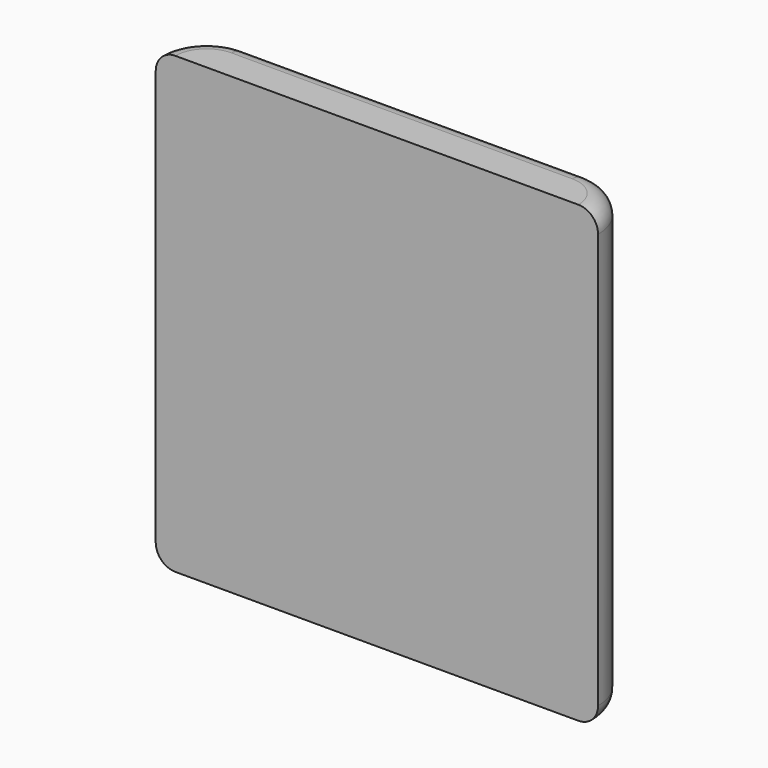
from build123d import *

# Parameters (mm, degrees)
F0_W         = 495.8
F0_H         = 57
F1_DEPTH     = 509.2
F2_R         = 56.99999
F3_T1_DEPTH  = 381.80002
F3_T3_DEPTH  = 55.00001
F3_T6_ANGLE  = 90
F3_T8_ANGLE  = 90
F3_T10_ANGLE = 90
F3_T12_ANGLE = 90


# Not quite as in the source:
# - a fillet or chamfer that OpenCascade refuses, or shapes differently, is made with other operations: its cross-section is extruded or revolved along the edge and cut away or added
# - a fillet or chamfer is up to 0.001 mm smaller than in the source, because OpenCascade refuses the exact size


with BuildPart() as f1:
    # F0 (on Top) → F1 (new body)
    with BuildSketch(Plane.XY):
        with Locations((247.9, 28.5)):
            Rectangle(F0_W, F0_H)
    extrude(amount=-F1_DEPTH)

    # F2 (radius 57 in the source; OpenCascade refuses exactly that, so slightly less here)
    f2_edges = [f1.edges().sort_by_distance(p)[0] for p in [
        (495.8, 57, -254.6),
        (0, 57, -254.6),
    ]]
    fillet(f2_edges, radius=F2_R)

    # F3: fillet of radius 22 on 6 edges, made by hand

    # F3_s2 → F3_t1 (cut)
    with BuildSketch(Plane.YZ.offset(56.99999)):
        with BuildLine():
            ThreePointArc((35, 0), (50.5563491861, -6.4436508139), (57, -22))
            Line((57, -22), (57, 0))
            Line((57, 0), (35, 0))
        make_face()
        with BuildLine():
            ThreePointArc((35, -509.2), (50.5563491861, -502.7563491861), (57, -487.2))
            Line((57, -487.2), (57, -509.2))
            Line((57, -509.2), (35, -509.2))
        make_face()
    extrude(amount=F3_T1_DEPTH, mode=Mode.SUBTRACT)

    # F3_s4 → F3_t3 (cut)
    with BuildSketch(Plane.XZ.offset(-1e-05)):
        with BuildLine():
            ThreePointArc((473.8, -509.2), (489.3563491861, -502.7563491861), (495.8, -487.2))
            Line((495.8, -487.2), (495.8, -509.2))
            Line((495.8, -509.2), (473.8, -509.2))
        make_face()
        with BuildLine():
            ThreePointArc((0, -487.2), (6.4436508139, -502.7563491861), (22, -509.2))
            Line((22, -509.2), (0, -509.2))
            Line((0, -509.2), (0, -487.2))
        make_face()
        with BuildLine():
            ThreePointArc((0, -22), (6.4436508139, -6.4436508139), (22, 0))
            Line((22, 0), (0, 0))
            Line((0, 0), (0, -22))
        make_face()
        with BuildLine():
            ThreePointArc((473.8, 0), (489.3563491861, -6.4436508139), (495.8, -22))
            Line((495.8, -22), (495.8, 0))
            Line((495.8, 0), (473.8, 0))
        make_face()
    extrude(amount=F3_T3_DEPTH, mode=Mode.SUBTRACT)

    # F3_s5 → F3_t6 (revolve, cut)
    with BuildSketch(Plane.XZ.offset(-1e-05)):
        with BuildLine():
            ThreePointArc((473.8, 0), (489.3563491861, -6.4436508139), (495.8, -22))
            Line((495.8, -22), (495.8, 0))
            Line((495.8, 0), (473.8, 0))
        make_face()
    revolve(axis=Axis((438.80001, 1e-05, 0), (0, 0, 1)), revolution_arc=F3_T6_ANGLE, mode=Mode.SUBTRACT)

    # F3_s7 → F3_t8 (revolve, cut)
    with BuildSketch(Plane.XZ.offset(-1e-05)):
        with BuildLine():
            ThreePointArc((22, 0), (6.4436508139, -6.4436508139), (0, -22))
            Line((0, -22), (0, 0))
            Line((0, 0), (22, 0))
        make_face()
    revolve(axis=Axis((56.99999, 1e-05, 0), (0, 0, -1)), revolution_arc=F3_T8_ANGLE, mode=Mode.SUBTRACT)

    # F3_s9 → F3_t10 (revolve, cut)
    with BuildSketch(Plane.XZ.offset(-1e-05)):
        with BuildLine():
            ThreePointArc((0, -487.2), (6.4436508139, -502.7563491861), (22, -509.2))
            Line((22, -509.2), (0, -509.2))
            Line((0, -509.2), (0, -487.2))
        make_face()
    revolve(axis=Axis((56.99999, 1e-05, -509.2), (0, 0, -1)), revolution_arc=F3_T10_ANGLE, mode=Mode.SUBTRACT)

    # F3_s11 → F3_t12 (revolve, cut)
    with BuildSketch(Plane.XZ.offset(-1e-05)):
        with BuildLine():
            ThreePointArc((473.8, -509.2), (489.3563491861, -502.7563491861), (495.8, -487.2))
            Line((495.8, -487.2), (495.8, -509.2))
            Line((495.8, -509.2), (473.8, -509.2))
        make_face()
    revolve(axis=Axis((438.80001, 1e-05, -509.2), (0, 0, 1)), revolution_arc=F3_T12_ANGLE, mode=Mode.SUBTRACT)


solid = f1.part
